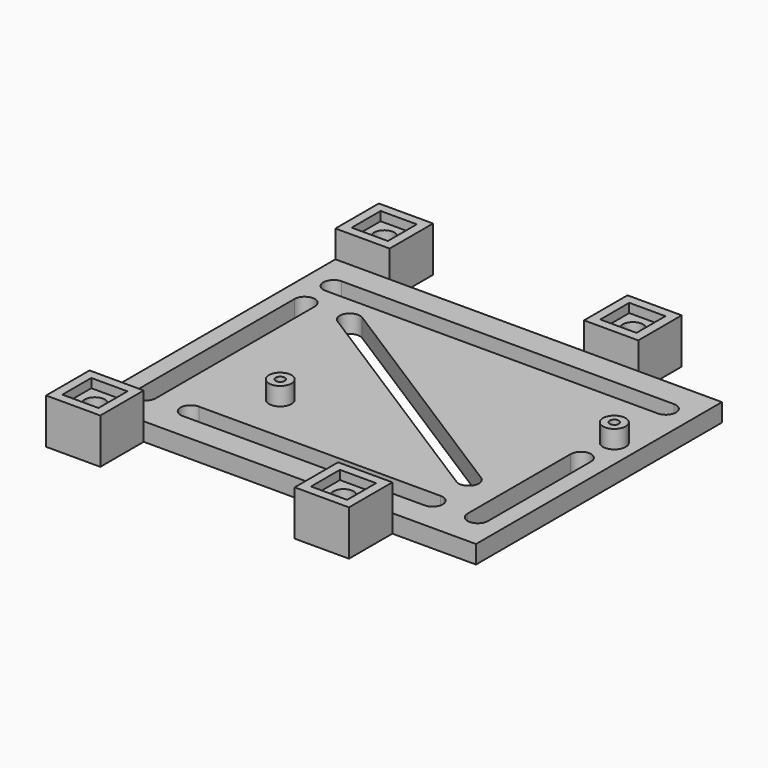
from build123d import *

# Parameters (mm, degrees)
F0_R      = 2.25
F0_R_2    = 1
F1_DEPTH  = 4
F2_W      = 12
F2_H      = 12
F2_R      = 2.25
F3_DEPTH  = 6
F4_W      = 8
F4_H      = 8
F4_R      = 2.25
F5_DEPTH  = 2
F6_R      = 4
F6_R_2    = 2.25
F7_DEPTH  = 5
F8_R      = 2.5
F8_R_2    = 1
F9_DEPTH  = 4
F11_DEPTH = 4.001


# Not quite as in the source:
# - a feature names something its author has since deleted; it is built from what else it names


with BuildPart() as f1:
    # F0 (on Top) → F1 (new body)
    with BuildSketch(Plane.XY):
        Polygon((-43.4, 46), (-55.4, 46), (-55.4, -46), (-43.4, -46), (-43.4, -34), (-0.4, -34), (-0.4, -46), (11.6, -46), (11.6, -34), (30.1, -34), (30.1, 34), (11.6, 34), (11.6, 46), (-0.4, 46), (-0.4, 34), (-43.4, 34), align=None)
        with Locations((-49.4, -40)):
            Circle(F0_R, mode=Mode.SUBTRACT)
        with Locations((-30, -13)):
            Circle(F0_R_2, mode=Mode.SUBTRACT)
        with Locations((5.6, -40)):
            Circle(F0_R, mode=Mode.SUBTRACT)
        with Locations((-49.4, 40)):
            Circle(F0_R, mode=Mode.SUBTRACT)
        with Locations((25.1, 10.5)):
            Circle(F0_R_2, mode=Mode.SUBTRACT)
        with Locations((5.6, 40)):
            Circle(F0_R, mode=Mode.SUBTRACT)
    extrude(amount=F1_DEPTH)

    # F2 (on face) → F3 (join)
    with BuildSketch(Plane.XY.offset(4)):
        with Locations((-49.4, -40)):
            Rectangle(F2_W, F2_H)
        with Locations((-49.4, -40)):
            Circle(F2_R, mode=Mode.SUBTRACT)
        with Locations((-49.4, 40)):
            Rectangle(F2_W, F2_H)
        with Locations((-49.4, 40)):
            Circle(F2_R, mode=Mode.SUBTRACT)
        with Locations((5.6, 40)):
            Rectangle(F2_W, F2_H)
        with Locations((5.6, 40)):
            Circle(F2_R, mode=Mode.SUBTRACT)
        with Locations((5.6, -40)):
            Rectangle(F2_W, F2_H)
        with Locations((5.6, -40)):
            Circle(F2_R, mode=Mode.SUBTRACT)
    extrude(amount=F3_DEPTH)

    # F4 (on face) → F5 (cut)
    with BuildSketch(Plane.XY.offset(10)):
        with Locations((-49.4, 40)):
            Rectangle(F4_W, F4_H)
        with Locations((-49.4, 40)):
            Circle(F4_R, mode=Mode.SUBTRACT)
        with Locations((5.6, 40)):
            Rectangle(F4_W, F4_H)
        with Locations((5.6, 40)):
            Circle(F4_R, mode=Mode.SUBTRACT)
        with Locations((5.6, -40)):
            Rectangle(F4_W, F4_H)
        with Locations((5.6, -40)):
            Circle(F4_R, mode=Mode.SUBTRACT)
        with Locations((-49.4, -40)):
            Rectangle(F4_W, F4_H)
        with Locations((-49.4, -40)):
            Circle(F4_R, mode=Mode.SUBTRACT)
    extrude(amount=-F5_DEPTH, mode=Mode.SUBTRACT)

    # F6 (on face) → F7 (cut)
    with BuildSketch(Plane(origin=(0, 0, 0), x_dir=(1, 0, 0), z_dir=(0, 0, -1))):
        with Locations((-49.4, 40)):
            Circle(F6_R)
        with Locations((-49.4, 40)):
            Circle(F6_R_2, mode=Mode.SUBTRACT)
        with Locations((5.6, 40)):
            Circle(F6_R)
        with Locations((5.6, 40)):
            Circle(F6_R_2, mode=Mode.SUBTRACT)
        with Locations((5.6, -40)):
            Circle(F6_R)
        with Locations((5.6, -40)):
            Circle(F6_R_2, mode=Mode.SUBTRACT)
        with Locations((-49.4, -40)):
            Circle(F6_R)
        with Locations((-49.4, -40)):
            Circle(F6_R_2, mode=Mode.SUBTRACT)
    extrude(amount=-F7_DEPTH, mode=Mode.SUBTRACT)

    # F8 (on face) → F9 (join)
    with BuildSketch(Plane.XY.offset(4)):
        with Locations((-30, -13)):
            Circle(F8_R)
        with Locations((-30, -13)):
            Circle(F8_R_2, mode=Mode.SUBTRACT)
        with Locations((25.1, 10.5)):
            Circle(F8_R)
        with Locations((25.1, 10.5)):
            Circle(F8_R_2, mode=Mode.SUBTRACT)
    extrude(amount=F9_DEPTH)

    # F10 (on face) → F11 (cut, through all)
    with BuildSketch(Plane.XY.offset(4)):
        with BuildLine():
            ThreePointArc((-49.4, 28.25), (-47.8090097423, 27.5909902577), (-47.15, 26))
            ThreePointArc((-47.15, 26), (-47.8090097423, 24.4090097423), (-49.4, 23.75))
            Line((-49.4, 23.75), (24.1, 23.75))
            ThreePointArc((24.1, 23.75), (21.85, 26), (24.1, 28.25))
            Line((24.1, 28.25), (-49.4, 28.25))
        make_face()
        with BuildLine():
            ThreePointArc((-49.4, 23.75), (-47.8090097423, 24.4090097423), (-47.15, 26))
            ThreePointArc((-47.15, 26), (-47.8090097423, 27.5909902577), (-49.4, 28.25))
            ThreePointArc((-49.4, 28.25), (-51.65, 26), (-49.4, 23.75))
        make_face()
        with BuildLine():
            Line((-47.15, -26), (-47.15, 18))
            ThreePointArc((-47.15, 18), (-49.4, 15.75), (-51.65, 18))
            Line((-51.65, 18), (-51.65, -26))
            ThreePointArc((-51.65, -26), (-49.4, -23.75), (-47.15, -26))
        make_face()
        with BuildLine():
            ThreePointArc((-51.65, 18), (-49.4, 15.75), (-47.15, 18))
            ThreePointArc((-47.15, 18), (-49.4, 20.25), (-51.65, 18))
        make_face()
        with BuildLine():
            ThreePointArc((-40.606821277, 16.1010312258), (-38.3166828427, 16.0279645194), (-37.15, 18))
            ThreePointArc((-37.15, 18), (-37.4279645194, 19.0833171573), (-38.193178723, 19.8989687742))
            ThreePointArc((-38.193178723, 19.8989687742), (-41.2989687742, 19.206821277), (-40.606821277, 16.1010312258))
        make_face()
        with BuildLine():
            ThreePointArc((-51.65, -26), (-49.4, -28.25), (-47.15, -26))
            ThreePointArc((-47.15, -26), (-49.4, -23.75), (-51.65, -26))
        make_face()
        with BuildLine():
            ThreePointArc((-39.4, -28.25), (-37.8090097423, -27.5909902577), (-37.15, -26))
            ThreePointArc((-37.15, -26), (-37.8090097423, -24.4090097423), (-39.4, -23.75))
            ThreePointArc((-39.4, -23.75), (-41.65, -26), (-39.4, -28.25))
        make_face()
        with BuildLine():
            ThreePointArc((-39.4, -23.75), (-37.8090097423, -24.4090097423), (-37.15, -26))
            ThreePointArc((-37.15, -26), (-37.8090097423, -27.5909902577), (-39.4, -28.25))
            Line((-39.4, -28.25), (14.1, -28.25))
            ThreePointArc((14.1, -28.25), (11.85, -26), (14.1, -23.75))
            Line((14.1, -23.75), (-39.4, -23.75))
        make_face()
        with BuildLine():
            ThreePointArc((16.35, -26), (15.6909902577, -24.4090097423), (14.1, -23.75))
            ThreePointArc((14.1, -23.75), (11.85, -26), (14.1, -28.25))
            ThreePointArc((14.1, -28.25), (15.6909902577, -27.5909902577), (16.35, -26))
        make_face()
        with BuildLine():
            ThreePointArc((21.85, -26), (24.1, -28.25), (26.35, -26))
            ThreePointArc((26.35, -26), (24.1, -23.75), (21.85, -26))
        make_face()
        with BuildLine():
            ThreePointArc((16.35, -16), (16.0720354806, -14.9166828427), (15.306821277, -14.1010312258))
            ThreePointArc((15.306821277, -14.1010312258), (12.2010312258, -14.793178723), (12.893178723, -17.8989687742))
            ThreePointArc((12.893178723, -17.8989687742), (15.1833171573, -17.9720354806), (16.35, -16))
        make_face()
        with BuildLine():
            ThreePointArc((-38.193178723, 19.8989687742), (-37.4279645194, 19.0833171573), (-37.15, 18))
            ThreePointArc((-37.15, 18), (-38.3166828427, 16.0279645194), (-40.606821277, 16.1010312258))
            Line((-40.606821277, 16.1010312258), (12.893178723, -17.8989687742))
            ThreePointArc((12.893178723, -17.8989687742), (12.2010312258, -14.793178723), (15.306821277, -14.1010312258))
            Line((15.306821277, -14.1010312258), (-38.193178723, 19.8989687742))
        make_face()
        with BuildLine():
            ThreePointArc((21.85, -26), (24.1, -23.75), (26.35, -26))
            Line((26.35, -26), (26.35, 2.5))
            ThreePointArc((26.35, 2.5), (24.1, 0.25), (21.85, 2.5))
            Line((21.85, 2.5), (21.85, -26))
        make_face()
        with BuildLine():
            ThreePointArc((21.85, 2.5), (24.1, 0.25), (26.35, 2.5))
            ThreePointArc((26.35, 2.5), (24.1, 4.75), (21.85, 2.5))
        make_face()
        with BuildLine():
            ThreePointArc((26.35, 26), (25.6909902577, 27.5909902577), (24.1, 28.25))
            ThreePointArc((24.1, 28.25), (21.85, 26), (24.1, 23.75))
            ThreePointArc((24.1, 23.75), (25.6909902577, 24.4090097423), (26.35, 26))
        make_face()
    extrude(amount=-F11_DEPTH, mode=Mode.SUBTRACT)


solid = f1.part
